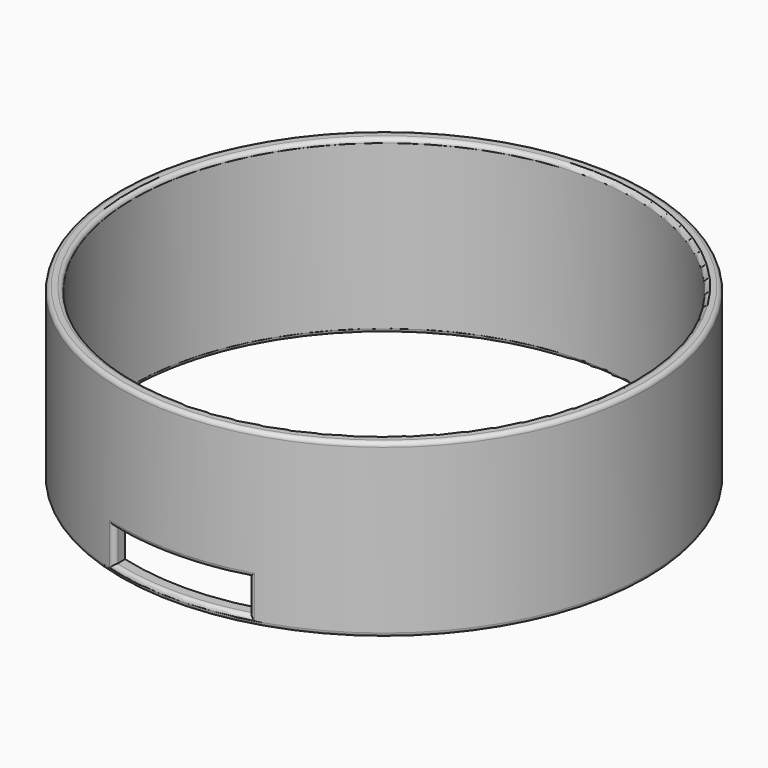
from build123d import *

# Parameters (mm, degrees)
F0_R         = 316.25
F1_DEPTH     = 205.7
F2_R         = 300
F3_DEPTH     = 631
F5_W         = 160
F5_H         = 40
F6_DEPTH     = 796.1248755455
F7_T1_DEPTH  = 40
F7_T10_ANGLE = 33.8359646931
F7_T16_ANGLE = 33.8359646931
F7_T27_ANGLE = 33.8359646931
F7_T31_DEPTH = 56.5905669687
F7_T38_DEPTH = 56.399324286
F7_T42_ANGLE = 33.8359646931
F7_T49_ANGLE = 33.8359646931
F7_T53_DEPTH = 56.5905669687
F7_T60_ANGLE = 33.8359646931
F7_T64_DEPTH = 56.399324286


# Not quite as in the source:
# - a fillet or chamfer that OpenCascade refuses, or shapes differently, is made with other operations: its cross-section is extruded or revolved along the edge and cut away or added


with BuildPart() as f1:
    # F0 (on Top) → F1 (new body)
    with BuildSketch(Plane.XY):
        Circle(F0_R)
    extrude(amount=F1_DEPTH)

    # F2 (on face) → F3 (cut)
    with BuildSketch(Plane.XY.offset(205.7)):
        Circle(F2_R)
    extrude(amount=-F3_DEPTH, mode=Mode.SUBTRACT)

    # F5 (on offset) → F6 (cut)
    with BuildSketch(Plane.XZ.offset(645.5422639847)):
        with Locations((1.6928017139, 30.4630875368)):
            Rectangle(F5_W, F5_H)
    extrude(amount=-F6_DEPTH, mode=Mode.SUBTRACT)

    # F7: fillet of radius 5 on 8 edges, made by hand

    # F7_s2 → F7_t1 (cut)
    with BuildSketch(Plane.XY.offset(10.4630875368)):
        with BuildLine():
            ThreePointArc((88.0854571632, -303.7351061968), (83.6897430437, -302.9306742994), (81.6928017139, -298.9329701304))
            Line((81.6928017139, -298.9329701304), (81.6928017139, -305.5165276186))
            ThreePointArc((81.6928017139, -305.5165276186), (84.8938022614, -304.6425853974), (88.0854571632, -303.7351061968))
        make_face()
        with BuildLine():
            ThreePointArc((-84.6454665316, -304.7116792899), (-80.2815860528, -303.8747654151), (-78.3071982861, -299.8941033327))
            Line((-78.3071982861, -299.8941033327), (-78.3071982861, -306.401770877))
            ThreePointArc((-78.3071982861, -306.401770877), (-81.4807145599, -305.5731592513), (-84.6454665316, -304.7116792899))
        make_face()
    extrude(amount=F7_T1_DEPTH, mode=Mode.SUBTRACT)

    # F7_s3 → F7_t4 (revolve, cut)
    with BuildSketch(Plane.XZ):
        with BuildLine():
            ThreePointArc((316.25, 200.7), (314.7855339059, 204.2355339059), (311.25, 205.7))
            Line((311.25, 205.7), (316.25, 205.7))
            Line((316.25, 205.7), (316.25, 200.7))
        make_face()
    revolve(axis=Axis((0, 0, 205.7), (0, 0, 1)), mode=Mode.SUBTRACT)

    # F7_s5 → F7_t6 (revolve, cut)
    with BuildSketch(Plane.XZ):
        with BuildLine():
            ThreePointArc((305, 205.7), (301.4644660941, 204.2355339059), (300, 200.7))
            Line((300, 200.7), (300, 205.7))
            Line((300, 205.7), (305, 205.7))
        make_face()
    revolve(axis=Axis((0, 0, 205.7), (0, 0, 1)), mode=Mode.SUBTRACT)


with BuildPart() as f7_tool8:
    # F7_s9 → F7_t10 (revolve)
    with BuildSketch(Plane(origin=(0, 0, 0), x_dir=(0, 0, 1), z_dir=(0.9550976314, 0.2962912662, 0))):
        with BuildLine():
            ThreePointArc((55.4630875368, 316.25), (51.9275536309, 314.7855339059), (50.4630875368, 311.25))
            Line((50.4630875368, 311.25), (50.4630875368, 316.25))
            Line((50.4630875368, 316.25), (55.4630875368, 316.25))
        make_face()
    revolve(axis=Axis((0, 0, 50.4630875368), (0, 0, -1)), revolution_arc=F7_T10_ANGLE)

    split(bisect_by=Plane.YZ.offset(-78.3071982861), keep=Keep.TOP)

    split(bisect_by=Plane.YZ.offset(81.6928017139), keep=Keep.BOTTOM)


with BuildPart() as f1_1:
    add(f1.part)

    # F7_t7: cut F7_tool8
    add(f7_tool8.part, mode=Mode.SUBTRACT)


with BuildPart() as f7_tool14:
    # F7_s15 → F7_t16 (revolve)
    with BuildSketch(Plane(origin=(0, 0, 0), x_dir=(0, 0, 1), z_dir=(0.9550976314, 0.2962912662, 0))):
        with BuildLine():
            ThreePointArc((5.4630875368, 316.25), (8.9986214427, 314.7855339059), (10.4630875368, 311.25))
            Line((10.4630875368, 311.25), (10.4630875368, 316.25))
            Line((10.4630875368, 316.25), (5.4630875368, 316.25))
        make_face()
    revolve(axis=Axis((0, 0, 10.4630875368), (0, 0, -1)), revolution_arc=F7_T16_ANGLE)

    split(bisect_by=Plane.YZ.offset(81.6928017139), keep=Keep.BOTTOM)

    split(bisect_by=Plane.YZ.offset(-78.3071982861), keep=Keep.TOP)


with BuildPart() as f1_2:
    add(f1_1.part)

    # F7_t13: cut F7_tool14
    add(f7_tool14.part, mode=Mode.SUBTRACT)

    # F7_s19 → F7_t20 (revolve, cut)
    with BuildSketch(Plane.XZ):
        with BuildLine():
            ThreePointArc((316.25, 5), (314.7855339059, 1.4644660941), (311.25, 0))
            Line((311.25, 0), (316.25, 0))
            Line((316.25, 0), (316.25, 5))
        make_face()
    revolve(axis=Axis((0, 0, 0), (0, 0, 1)), mode=Mode.SUBTRACT)

    # F7_s21 → F7_t22 (revolve, cut)
    with BuildSketch(Plane.XZ):
        with BuildLine():
            ThreePointArc((305, 0), (301.4644660941, 1.4644660941), (300, 5))
            Line((300, 5), (300, 0))
            Line((300, 0), (305, 0))
        make_face()
    revolve(axis=Axis((0, 0, 0), (0, 0, 1)), mode=Mode.SUBTRACT)


with BuildPart() as f7_tool25:
    # F7_s26 → F7_t27 (revolve)
    with BuildSketch(Plane(origin=(0, 0, 0), x_dir=(0, 0, 1), z_dir=(0.9550976314, 0.2962912662, 0))):
        with BuildLine():
            ThreePointArc((55.4630875368, 316.25), (51.9275536309, 314.7855339059), (50.4630875368, 311.25))
            Line((50.4630875368, 311.25), (50.4630875368, 316.25))
            Line((50.4630875368, 316.25), (55.4630875368, 316.25))
        make_face()
    revolve(axis=Axis((0, 0, 50.4630875368), (0, 0, -1)), revolution_arc=F7_T27_ANGLE)

    split(bisect_by=Plane.YZ.offset(81.6928017139), keep=Keep.TOP)


with BuildPart() as f7_tool29:
    # F7_s30 → F7_t31 (new body)
    with BuildSketch(Plane.XY.offset(67.0536545055)):
        with BuildLine():
            ThreePointArc((88.0854571632, -303.7351061968), (83.6897430437, -302.9306742994), (81.6928017139, -298.9329701304))
            Line((81.6928017139, -298.9329701304), (81.6928017139, -305.5165276186))
            ThreePointArc((81.6928017139, -305.5165276186), (84.8938022614, -304.6425853974), (88.0854571632, -303.7351061968))
        make_face()
    extrude(amount=-F7_T31_DEPTH)

    split(bisect_by=Plane.XY.offset(50.4630875368), keep=Keep.TOP)


with BuildPart() as f7_tool25_1:
    add(f7_tool25.part)

    # F7_t33: intersect F7_tool29
    add(f7_tool29.part, mode=Mode.INTERSECT)


with BuildPart() as f1_3:
    add(f1_2.part)

    # F7_t23: cut F7_tool25
    add(f7_tool25_1.part, mode=Mode.SUBTRACT)


with BuildPart() as f7_tool36:
    # F7_s37 → F7_t38 (new body)
    with BuildSketch(Plane.XY.offset(66.8624118228)):
        with BuildLine():
            ThreePointArc((-84.6454665316, -304.7116792899), (-80.2815860528, -303.8747654151), (-78.3071982861, -299.8941033327))
            Line((-78.3071982861, -299.8941033327), (-78.3071982861, -306.401770877))
            ThreePointArc((-78.3071982861, -306.401770877), (-81.4807145599, -305.5731592513), (-84.6454665316, -304.7116792899))
        make_face()
    extrude(amount=-F7_T38_DEPTH)

    split(bisect_by=Plane.XY.offset(50.4630875368), keep=Keep.TOP)


with BuildPart() as f7_tool40:
    # F7_s41 → F7_t42 (revolve)
    with BuildSketch(Plane(origin=(0, 0, 0), x_dir=(0, 0, 1), z_dir=(0.9550976314, 0.2962912662, 0))):
        with BuildLine():
            ThreePointArc((55.4630875368, 316.25), (51.9275536309, 314.7855339059), (50.4630875368, 311.25))
            Line((50.4630875368, 311.25), (50.4630875368, 316.25))
            Line((50.4630875368, 316.25), (55.4630875368, 316.25))
        make_face()
    revolve(axis=Axis((0, 0, 50.4630875368), (0, 0, -1)), revolution_arc=F7_T42_ANGLE)

    split(bisect_by=Plane.YZ.offset(-78.3071982861), keep=Keep.BOTTOM)


with BuildPart() as f7_tool36_1:
    add(f7_tool36.part)

    # F7_t44: intersect F7_tool40
    add(f7_tool40.part, mode=Mode.INTERSECT)


with BuildPart() as f1_4:
    add(f1_3.part)

    # F7_t34: cut F7_tool36
    add(f7_tool36_1.part, mode=Mode.SUBTRACT)


with BuildPart() as f7_tool47:
    # F7_s48 → F7_t49 (revolve)
    with BuildSketch(Plane(origin=(0, 0, 0), x_dir=(0, 0, 1), z_dir=(0.9550976314, 0.2962912662, 0))):
        with BuildLine():
            ThreePointArc((5.4630875368, 316.25), (8.9986214427, 314.7855339059), (10.4630875368, 311.25))
            Line((10.4630875368, 311.25), (10.4630875368, 316.25))
            Line((10.4630875368, 316.25), (5.4630875368, 316.25))
        make_face()
    revolve(axis=Axis((0, 0, 10.4630875368), (0, 0, -1)), revolution_arc=F7_T49_ANGLE)

    split(bisect_by=Plane.YZ.offset(81.6928017139), keep=Keep.TOP)


with BuildPart() as f7_tool51:
    # F7_s52 → F7_t53 (new body)
    with BuildSketch(Plane.XY.offset(50.4630875368)):
        with BuildLine():
            ThreePointArc((88.0854571632, -303.7351061968), (83.6897430437, -302.9306742994), (81.6928017139, -298.9329701304))
            Line((81.6928017139, -298.9329701304), (81.6928017139, -305.5165276186))
            ThreePointArc((81.6928017139, -305.5165276186), (84.8938022614, -304.6425853974), (88.0854571632, -303.7351061968))
        make_face()
    extrude(amount=-F7_T53_DEPTH)

    split(bisect_by=Plane.XY.offset(10.4630875368), keep=Keep.BOTTOM)


with BuildPart() as f7_tool47_1:
    add(f7_tool47.part)

    # F7_t55: intersect F7_tool51
    add(f7_tool51.part, mode=Mode.INTERSECT)


with BuildPart() as f1_5:
    add(f1_4.part)

    # F7_t45: cut F7_tool47
    add(f7_tool47_1.part, mode=Mode.SUBTRACT)


with BuildPart() as f7_tool58:
    # F7_s59 → F7_t60 (revolve)
    with BuildSketch(Plane(origin=(0, 0, 0), x_dir=(0, 0, 1), z_dir=(0.9550976314, 0.2962912662, 0))):
        with BuildLine():
            ThreePointArc((5.4630875368, 316.25), (8.9986214427, 314.7855339059), (10.4630875368, 311.25))
            Line((10.4630875368, 311.25), (10.4630875368, 316.25))
            Line((10.4630875368, 316.25), (5.4630875368, 316.25))
        make_face()
    revolve(axis=Axis((0, 0, 10.4630875368), (0, 0, -1)), revolution_arc=F7_T60_ANGLE)

    split(bisect_by=Plane.YZ.offset(-78.3071982861), keep=Keep.BOTTOM)


with BuildPart() as f7_tool62:
    # F7_s63 → F7_t64 (new body)
    with BuildSketch(Plane.XY.offset(50.4630875368)):
        with BuildLine():
            ThreePointArc((-84.6454665316, -304.7116792899), (-80.2815860528, -303.8747654151), (-78.3071982861, -299.8941033327))
            Line((-78.3071982861, -299.8941033327), (-78.3071982861, -306.401770877))
            ThreePointArc((-78.3071982861, -306.401770877), (-81.4807145599, -305.5731592513), (-84.6454665316, -304.7116792899))
        make_face()
    extrude(amount=-F7_T64_DEPTH)

    split(bisect_by=Plane.XY.offset(10.4630875368), keep=Keep.BOTTOM)


with BuildPart() as f7_tool58_1:
    add(f7_tool58.part)

    # F7_t66: intersect F7_tool62
    add(f7_tool62.part, mode=Mode.INTERSECT)


with BuildPart() as f1_6:
    add(f1_5.part)

    # F7_t56: cut F7_tool58
    add(f7_tool58_1.part, mode=Mode.SUBTRACT)


solid = f1_6.part
